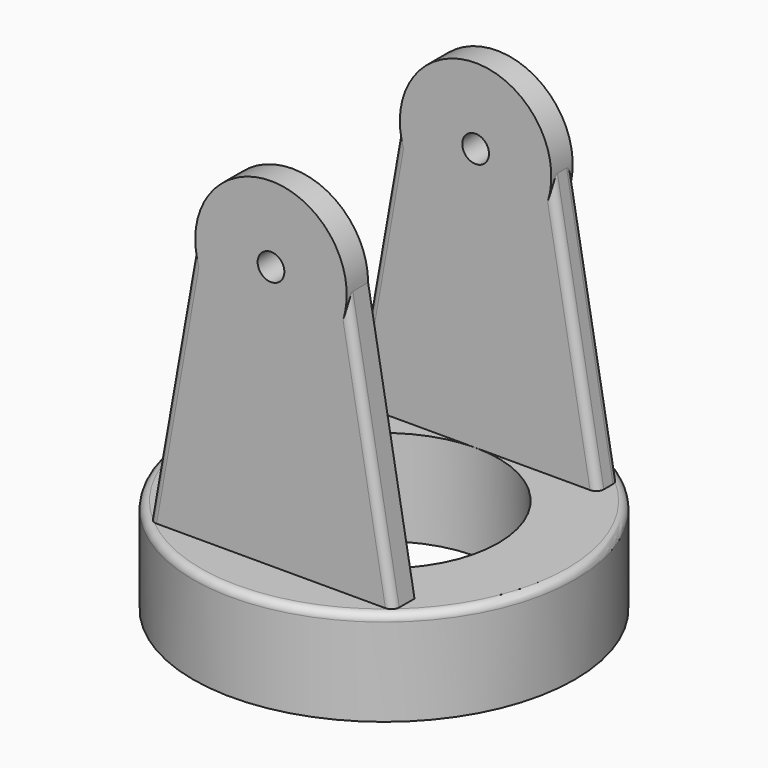
from build123d import *

# Parameters (mm, degrees)
F0_R          = 63.5
F0_R_2        = 38.1
F1_DEPTH      = 31.75
F4_DEPTH      = 8.89
F9_D          = 8.89
F11_DEPTH     = 8.89
F13_D         = 8.89
F14_T4_DEPTH  = 114.3
F14_S6_R      = 25.2026770054
F14_T7_DEPTH  = 59
F14_T11_DEPTH = 114.3
F14_S13_R     = 25.2026770054
F14_T14_DEPTH = 59
F14_T18_DEPTH = 114.3
F14_S20_R     = 25.2026770054
F14_T21_DEPTH = 59
F14_T25_DEPTH = 114.3
F14_S27_R     = 25.2026770054
F14_T28_DEPTH = 59
F14_T32_DEPTH = 114.3
F14_S34_R     = 25.2026770054
F14_T35_DEPTH = 59
F14_T39_DEPTH = 114.3
F14_S41_R     = 25.2026770054
F14_T42_DEPTH = 59
F14_T46_DEPTH = 114.3
F14_S48_R     = 25.2026770054
F14_T49_DEPTH = 59
F14_S54_R     = 2.54
F14_T55_DEPTH = 99
F14_S56_R     = 2.54
F14_T57_DEPTH = 99


# Not quite as in the source:
# - a fillet or chamfer that OpenCascade refuses, or shapes differently, is made with other operations: its cross-section is extruded or revolved along the edge and cut away or added
# - a feature of the source that left no trace in its solid (it failed there, or was rolled back) is left out


with BuildPart() as f1:
    # F0 (on Top) → F1 (new body)
    with BuildSketch(Plane.XY):
        Circle(F0_R)
        Circle(F0_R_2, mode=Mode.SUBTRACT)
    extrude(amount=F1_DEPTH)

    # F3 (on offset) → F4 (join)
    with BuildSketch(Plane.XZ.offset(38.1)):
        with BuildLine():
            Line((-25.2026770054, 119.2994092428), (-40.64, 31.75))
            Line((-40.64, 31.75), (40.64, 31.75))
            Line((40.64, 31.75), (25.2026770054, 119.2994092428))
            ThreePointArc((25.2026770054, 119.2994092428), (0, 144.5020862482), (-25.2026770054, 119.2994092428))
        make_face()
    extrude(amount=F4_DEPTH)

    # F9 (through all)
    with Locations(Plane.XZ.offset(46.99)):
        with Locations((0, 119.2994092428)):
            Hole(F9_D / 2)

    # F6 (on offset) → F11 (join)
    with BuildSketch(Plane.XZ.offset(-38.1)):
        with BuildLine():
            Line((-25.2026770054, 119.2994092428), (-40.64, 31.75))
            Line((-40.64, 31.75), (40.64, 31.75))
            Line((40.64, 31.75), (25.2026770054, 119.2994092428))
            ThreePointArc((25.2026770054, 119.2994092428), (0, 144.5020862482), (-25.2026770054, 119.2994092428))
        make_face()
    extrude(amount=-F11_DEPTH)

    # F13 (through all)
    with Locations(Plane(origin=(0, 46.99, 0), x_dir=(-1, 0, 0), z_dir=(0, 1, 0))):
        with Locations((0, 119.2994092428)):
            Hole(F13_D / 2)

    # F14: fillet of radius 2.54 on 8 edges, made by hand


with BuildPart() as f14_tool2:
    # F14_s3 → F14_t4 (new body)
    with BuildSketch(Plane(origin=(22.9494446088, 0, 130.1527679803), x_dir=(0, 1, 0), z_dir=(-0.1736481777, 0, -0.984807753))):
        with BuildLine():
            ThreePointArc((-46.99, -42.9959167233), (-46.2460512242, -44.7919679476), (-44.45, -45.5359167233))
            Line((-44.45, -45.5359167233), (-46.99, -45.5359167233))
            Line((-46.99, -45.5359167233), (-46.99, -42.9959167233))
        make_face()
    extrude(amount=F14_T4_DEPTH)

    split(bisect_by=Plane.XY.offset(31.75), keep=Keep.TOP)

    # F14_s6 → F14_t7 (cut, symmetric)
    with BuildSketch(Plane.XZ.offset(45.7)):
        with Locations((0, 119.2994092428)):
            Circle(F14_S6_R)
    extrude(amount=F14_T7_DEPTH, both=True, mode=Mode.SUBTRACT)


with BuildPart() as f1_1:
    add(f1.part)

    # F14_t1: cut F14_tool2
    add(f14_tool2.part, mode=Mode.SUBTRACT)


with BuildPart() as f14_tool9:
    # F14_s10 → F14_t11 (new body)
    with BuildSketch(Plane(origin=(-3.1014579015, 0, 17.589241811), x_dir=(0, 1, 0), z_dir=(-0.1736481777, 0, 0.984807753))):
        with BuildLine():
            ThreePointArc((-46.99, -42.9959167233), (-46.2460512242, -44.7919679476), (-44.45, -45.5359167233))
            Line((-44.45, -45.5359167233), (-46.99, -45.5359167233))
            Line((-46.99, -45.5359167233), (-46.99, -42.9959167233))
        make_face()
    extrude(amount=F14_T11_DEPTH)

    split(bisect_by=Plane.XY.offset(31.75), keep=Keep.TOP)

    # F14_s13 → F14_t14 (cut, symmetric)
    with BuildSketch(Plane.XZ.offset(45.7)):
        with Locations((0, 119.2994092428)):
            Circle(F14_S13_R)
    extrude(amount=F14_T14_DEPTH, both=True, mode=Mode.SUBTRACT)


with BuildPart() as f1_2:
    add(f1_1.part)

    # F14_t8: cut F14_tool9
    add(f14_tool9.part, mode=Mode.SUBTRACT)


with BuildPart() as f14_tool16:
    # F14_s17 → F14_t18 (new body)
    with BuildSketch(Plane(origin=(22.9494446088, 0, 130.1527679803), x_dir=(0, 1, 0), z_dir=(-0.1736481777, 0, -0.984807753))):
        with BuildLine():
            ThreePointArc((-40.64, -45.5359167233), (-38.8439487758, -44.7919679476), (-38.1, -42.9959167233))
            Line((-38.1, -42.9959167233), (-38.1, -45.5359167233))
            Line((-38.1, -45.5359167233), (-40.64, -45.5359167233))
        make_face()
    extrude(amount=F14_T18_DEPTH)

    split(bisect_by=Plane.XY.offset(31.75), keep=Keep.TOP)

    # F14_s20 → F14_t21 (cut, symmetric)
    with BuildSketch(Plane.XZ.offset(39.4)):
        with Locations((0, 119.2994092428)):
            Circle(F14_S20_R)
    extrude(amount=F14_T21_DEPTH, both=True, mode=Mode.SUBTRACT)


with BuildPart() as f1_3:
    add(f1_2.part)

    # F14_t15: cut F14_tool16
    add(f14_tool16.part, mode=Mode.SUBTRACT)


with BuildPart() as f14_tool23:
    # F14_s24 → F14_t25 (new body)
    with BuildSketch(Plane(origin=(-3.1014579015, 0, 17.589241811), x_dir=(0, 1, 0), z_dir=(-0.1736481777, 0, 0.984807753))):
        with BuildLine():
            ThreePointArc((40.64, -45.5359167233), (38.8439487758, -44.7919679476), (38.1, -42.9959167233))
            Line((38.1, -42.9959167233), (38.1, -45.5359167233))
            Line((38.1, -45.5359167233), (40.64, -45.5359167233))
        make_face()
    extrude(amount=F14_T25_DEPTH)

    split(bisect_by=Plane.XY.offset(31.75), keep=Keep.TOP)

    # F14_s27 → F14_t28 (cut, symmetric)
    with BuildSketch(Plane.XZ.offset(-39.4)):
        with Locations((0, 119.2994092428)):
            Circle(F14_S27_R)
    extrude(amount=F14_T28_DEPTH, both=True, mode=Mode.SUBTRACT)


with BuildPart() as f1_4:
    add(f1_3.part)

    # F14_t22: cut F14_tool23
    add(f14_tool23.part, mode=Mode.SUBTRACT)


with BuildPart() as f14_tool30:
    # F14_s31 → F14_t32 (new body)
    with BuildSketch(Plane(origin=(-3.1014579015, 0, 17.589241811), x_dir=(0, 1, 0), z_dir=(-0.1736481777, 0, 0.984807753))):
        with BuildLine():
            ThreePointArc((44.45, -45.5359167233), (46.2460512242, -44.7919679476), (46.99, -42.9959167233))
            Line((46.99, -42.9959167233), (46.99, -45.5359167233))
            Line((46.99, -45.5359167233), (44.45, -45.5359167233))
        make_face()
    extrude(amount=F14_T32_DEPTH)

    split(bisect_by=Plane.XY.offset(31.75), keep=Keep.TOP)

    # F14_s34 → F14_t35 (cut, symmetric)
    with BuildSketch(Plane.XZ.offset(-45.7)):
        with Locations((0, 119.2994092428)):
            Circle(F14_S34_R)
    extrude(amount=F14_T35_DEPTH, both=True, mode=Mode.SUBTRACT)


with BuildPart() as f1_5:
    add(f1_4.part)

    # F14_t29: cut F14_tool30
    add(f14_tool30.part, mode=Mode.SUBTRACT)


with BuildPart() as f14_tool37:
    # F14_s38 → F14_t39 (new body)
    with BuildSketch(Plane(origin=(22.9494446088, 0, 130.1527679803), x_dir=(0, 1, 0), z_dir=(-0.1736481777, 0, -0.984807753))):
        with BuildLine():
            ThreePointArc((46.99, -42.9959167233), (46.2460512242, -44.7919679476), (44.45, -45.5359167233))
            Line((44.45, -45.5359167233), (46.99, -45.5359167233))
            Line((46.99, -45.5359167233), (46.99, -42.9959167233))
        make_face()
    extrude(amount=F14_T39_DEPTH)

    split(bisect_by=Plane.XY.offset(31.75), keep=Keep.TOP)

    # F14_s41 → F14_t42 (cut, symmetric)
    with BuildSketch(Plane.XZ.offset(-45.7)):
        with Locations((0, 119.2994092428)):
            Circle(F14_S41_R)
    extrude(amount=F14_T42_DEPTH, both=True, mode=Mode.SUBTRACT)


with BuildPart() as f1_6:
    add(f1_5.part)

    # F14_t36: cut F14_tool37
    add(f14_tool37.part, mode=Mode.SUBTRACT)


with BuildPart() as f14_tool44:
    # F14_s45 → F14_t46 (new body)
    with BuildSketch(Plane(origin=(22.9494446088, 0, 130.1527679803), x_dir=(0, 1, 0), z_dir=(-0.1736481777, 0, -0.984807753))):
        with BuildLine():
            ThreePointArc((40.64, -45.5359167233), (38.8439487758, -44.7919679476), (38.1, -42.9959167233))
            Line((38.1, -42.9959167233), (38.1, -45.5359167233))
            Line((38.1, -45.5359167233), (40.64, -45.5359167233))
        make_face()
    extrude(amount=F14_T46_DEPTH)

    split(bisect_by=Plane.XY.offset(31.75), keep=Keep.TOP)

    # F14_s48 → F14_t49 (cut, symmetric)
    with BuildSketch(Plane.XZ.offset(-39.4)):
        with Locations((0, 119.2994092428)):
            Circle(F14_S48_R)
    extrude(amount=F14_T49_DEPTH, both=True, mode=Mode.SUBTRACT)


with BuildPart() as f1_7:
    add(f1_6.part)

    # F14_t43: cut F14_tool44
    add(f14_tool44.part, mode=Mode.SUBTRACT)


with BuildPart() as f14_tool51:
    # F14_s52 → F14_t53 (revolve)
    with BuildSketch(Plane.XZ):
        with BuildLine():
            ThreePointArc((63.5, 29.21), (62.7560512242, 31.0060512242), (60.96, 31.75))
            Line((60.96, 31.75), (63.5, 31.75))
            Line((63.5, 31.75), (63.5, 29.21))
        make_face()
    revolve(axis=Axis((0, 0, 31.75), (0, 0, 1)))

    # F14_s54 → F14_t55 (cut, symmetric)
    with BuildSketch(Plane(origin=(5.20944533, 0, 29.5442325904), x_dir=(0, 1, 0), z_dir=(0.1736481777, 0, 0.984807753))):
        with Locations((-44.45, 42.9959167233)):
            Circle(F14_S54_R)
    extrude(amount=F14_T55_DEPTH, both=True, mode=Mode.SUBTRACT)

    # F14_s56 → F14_t57 (cut, symmetric)
    with BuildSketch(Plane(origin=(-5.20944533, 0, 29.5442325904), x_dir=(0, 1, 0), z_dir=(0.1736481777, 0, -0.984807753))):
        with Locations((-44.45, 42.9959167233)):
            Circle(F14_S56_R)
    extrude(amount=F14_T57_DEPTH, both=True, mode=Mode.SUBTRACT)


with BuildPart() as f1_8:
    add(f1_7.part)

    # F14_t50: cut F14_tool51
    add(f14_tool51.part, mode=Mode.SUBTRACT)


solid = f1_8.part
